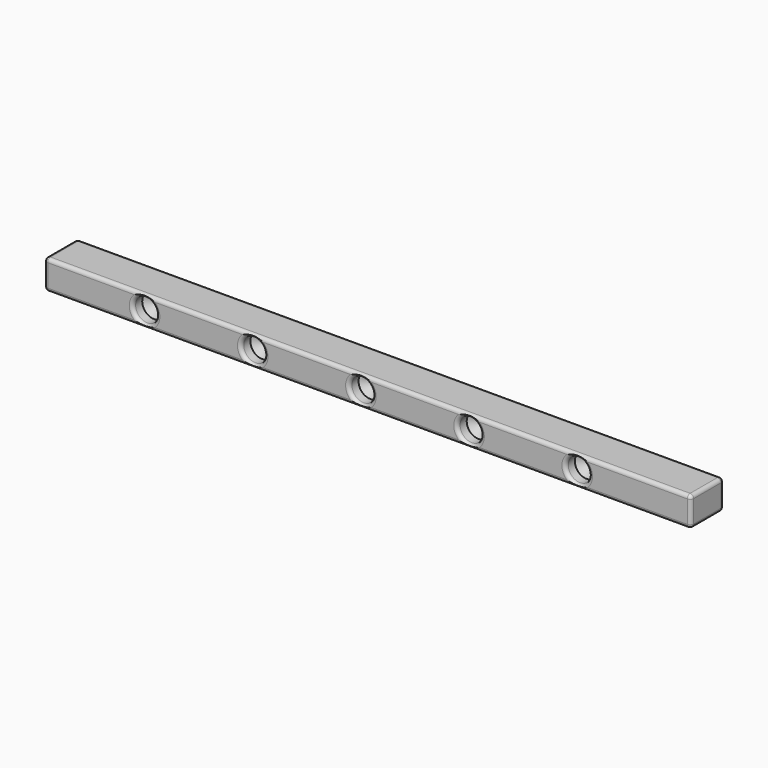
from build123d import *

# Parameters (mm, degrees)
F0_W         = 550
F0_H         = 25
F1_DEPTH     = 35
F3_D         = 20
F3_DEPTH     = 10
F3_TIP       = 6.0086061903
F4_T1_DEPTH  = 544
F4_T3_DEPTH  = 19
F4_T5_DEPTH  = 29
F4_S9_W      = 3
F4_S9_H      = 3
F4_T10_DEPTH = 3
F4_S15_W     = 3
F4_S15_H     = 3
F4_T16_DEPTH = 3
F4_S21_W     = 3
F4_S21_H     = 3
F4_T22_DEPTH = 3
F4_S27_W     = 3
F4_S27_H     = 3
F4_T28_DEPTH = 3
F4_S33_W     = 3
F4_S33_H     = 3
F4_T34_DEPTH = 3
F4_S39_W     = 3
F4_S39_H     = 3
F4_T40_DEPTH = 3
F4_S45_W     = 3
F4_S45_H     = 3
F4_T46_DEPTH = 3
F4_S51_W     = 3
F4_S51_H     = 3
F4_T52_DEPTH = 3


# Not quite as in the source:
# - a fillet or chamfer that OpenCascade refuses, or shapes differently, is made with other operations: its cross-section is extruded or revolved along the edge and cut away or added
# - a feature names something its author has since deleted; it is built from what else it names


with BuildPart() as f1:
    # F0 (on Front) → F1 (new body)
    with BuildSketch(Plane.XZ):
        with Locations((5.6565068662, -12.5)):
            Rectangle(F0_W, F0_H)
    extrude(amount=-F1_DEPTH)

    # F3
    with Locations(Plane.XZ):
        with Locations((0, -12.5), (-92, -12.5), (-184, -12.5), (92, -12.5), (184, -12.5)):
            Hole(F3_D / 2, depth=F3_DEPTH)
            with Locations((0, 0, -(F3_DEPTH + F3_TIP / 2))):  # 118° drill point
                Cone(0, F3_D / 2, F3_TIP, mode=Mode.SUBTRACT)

    # F4: fillet of radius 3 on 17 edges, made by hand

    # F4_s2 → F4_t1 (cut)
    with BuildSketch(Plane.YZ.offset(-266.3434931338)):
        with BuildLine():
            ThreePointArc((32, 0), (34.1213203436, -0.8786796564), (35, -3))
            Line((35, -3), (35, 0))
            Line((35, 0), (32, 0))
        make_face()
        with BuildLine():
            ThreePointArc((35, -22), (34.1213203436, -24.1213203436), (32, -25))
            Line((32, -25), (35, -25))
            Line((35, -25), (35, -22))
        make_face()
        with BuildLine():
            ThreePointArc((3, 0), (0.8786796564, -0.8786796564), (0, -3))
            Line((0, -3), (0, 0))
            Line((0, 0), (3, 0))
        make_face()
        with BuildLine():
            ThreePointArc((0, -22), (0.8786796564, -24.1213203436), (3, -25))
            Line((3, -25), (0, -25))
            Line((0, -25), (0, -22))
        make_face()
    extrude(amount=F4_T1_DEPTH, mode=Mode.SUBTRACT)

    # F4_s4 → F4_t3 (cut)
    with BuildSketch(Plane.XY.offset(-22)):
        with BuildLine():
            ThreePointArc((-269.3434931338, 32), (-268.4648134773, 34.1213203436), (-266.3434931338, 35))
            Line((-266.3434931338, 35), (-269.3434931338, 35))
            Line((-269.3434931338, 35), (-269.3434931338, 32))
        make_face()
        with BuildLine():
            ThreePointArc((280.6565068662, 32), (279.7778272098, 34.1213203436), (277.6565068662, 35))
            Line((277.6565068662, 35), (280.6565068662, 35))
            Line((280.6565068662, 35), (280.6565068662, 32))
        make_face()
        with BuildLine():
            ThreePointArc((280.6565068662, 3), (279.7778272098, 0.8786796564), (277.6565068662, 0))
            Line((277.6565068662, 0), (280.6565068662, 0))
            Line((280.6565068662, 0), (280.6565068662, 3))
        make_face()
        with BuildLine():
            ThreePointArc((-269.3434931338, 3), (-268.4648134773, 0.8786796564), (-266.3434931338, 0))
            Line((-266.3434931338, 0), (-269.3434931338, 0))
            Line((-269.3434931338, 0), (-269.3434931338, 3))
        make_face()
    extrude(amount=F4_T3_DEPTH, mode=Mode.SUBTRACT)

    # F4_s6 → F4_t5 (cut)
    with BuildSketch(Plane.XZ.offset(-32)):
        with BuildLine():
            ThreePointArc((280.6565068662, -22), (279.7778272098, -24.1213203436), (277.6565068662, -25))
            Line((277.6565068662, -25), (280.6565068662, -25))
            Line((280.6565068662, -25), (280.6565068662, -22))
        make_face()
        with BuildLine():
            ThreePointArc((277.6565068662, 0), (279.7778272098, -0.8786796564), (280.6565068662, -3))
            Line((280.6565068662, -3), (280.6565068662, 0))
            Line((280.6565068662, 0), (277.6565068662, 0))
        make_face()
        with BuildLine():
            ThreePointArc((-266.3434931338, 0), (-268.4648134773, -0.8786796564), (-269.3434931338, -3))
            Line((-269.3434931338, -3), (-269.3434931338, 0))
            Line((-269.3434931338, 0), (-266.3434931338, 0))
        make_face()
        with BuildLine():
            ThreePointArc((-269.3434931338, -22), (-268.4648134773, -24.1213203436), (-266.3434931338, -25))
            Line((-266.3434931338, -25), (-269.3434931338, -25))
            Line((-269.3434931338, -25), (-269.3434931338, -22))
        make_face()
    extrude(amount=F4_T5_DEPTH, mode=Mode.SUBTRACT)


with BuildPart() as f4_tool8:
    # F4_s9 → F4_t10 (new body)
    with BuildSketch(Plane.XY.offset(-3)):
        with Locations((279.1565068662, 33.5)):
            Rectangle(F4_S9_W, F4_S9_H)
    extrude(amount=F4_T10_DEPTH)

    # F4_s11 → F4_t12 (revolve, cut)
    with BuildSketch(Plane(origin=(277.6565068662, 32, -3), x_dir=(-0.7071067812, -0.7071067812, 0), z_dir=(-0.7071067812, 0.7071067812, 0))):
        with BuildLine():
            ThreePointArc((0, -3), (3, 0), (0, 3))
            Line((0, 3), (0, -3))
        make_face()
    revolve(axis=Axis((277.6565068662, 32, -3), (0, 0, 1)), mode=Mode.SUBTRACT)


with BuildPart() as f1_1:
    add(f1.part)

    # F4_t7: cut F4_tool8
    add(f4_tool8.part, mode=Mode.SUBTRACT)


with BuildPart() as f4_tool14:
    # F4_s15 → F4_t16 (new body)
    with BuildSketch(Plane.XY.offset(-3)):
        with Locations((-267.8434931338, 33.5)):
            Rectangle(F4_S15_W, F4_S15_H)
    extrude(amount=F4_T16_DEPTH)

    # F4_s17 → F4_t18 (revolve, cut)
    with BuildSketch(Plane(origin=(-266.3434931338, 32, -3), x_dir=(0.7071067812, -0.7071067812, 0), z_dir=(-0.7071067812, -0.7071067812, 0))):
        with BuildLine():
            ThreePointArc((0, -3), (3, 0), (0, 3))
            Line((0, 3), (0, -3))
        make_face()
    revolve(axis=Axis((-266.3434931338, 32, -3), (0, 0, 1)), mode=Mode.SUBTRACT)


with BuildPart() as f1_2:
    add(f1_1.part)

    # F4_t13: cut F4_tool14
    add(f4_tool14.part, mode=Mode.SUBTRACT)


with BuildPart() as f4_tool20:
    # F4_s21 → F4_t22 (new body)
    with BuildSketch(Plane.YZ.offset(-266.3434931338)):
        with Locations((33.5, -23.5)):
            Rectangle(F4_S21_W, F4_S21_H)
    extrude(amount=-F4_T22_DEPTH)

    # F4_s23 → F4_t24 (revolve, cut)
    with BuildSketch(Plane(origin=(-266.3434931338, 32, -22), x_dir=(0, -0.7071067812, 0.7071067812), z_dir=(0, -0.7071067812, -0.7071067812))):
        with BuildLine():
            ThreePointArc((0, -3), (3, 0), (0, 3))
            Line((0, 3), (0, -3))
        make_face()
    revolve(axis=Axis((-266.3434931338, 32, -22), (-1, 0, 0)), mode=Mode.SUBTRACT)


with BuildPart() as f1_3:
    add(f1_2.part)

    # F4_t19: cut F4_tool20
    add(f4_tool20.part, mode=Mode.SUBTRACT)


with BuildPart() as f4_tool26:
    # F4_s27 → F4_t28 (new body)
    with BuildSketch(Plane.YZ.offset(277.6565068662)):
        with Locations((33.5, -23.5)):
            Rectangle(F4_S27_W, F4_S27_H)
    extrude(amount=F4_T28_DEPTH)

    # F4_s29 → F4_t30 (revolve, cut)
    with BuildSketch(Plane(origin=(277.6565068662, 32, -22), x_dir=(0, -0.7071067812, 0.7071067812), z_dir=(0, 0.7071067812, 0.7071067812))):
        with BuildLine():
            ThreePointArc((0, -3), (3, 0), (0, 3))
            Line((0, 3), (0, -3))
        make_face()
    revolve(axis=Axis((277.6565068662, 32, -22), (1, 0, 0)), mode=Mode.SUBTRACT)


with BuildPart() as f1_4:
    add(f1_3.part)

    # F4_t25: cut F4_tool26
    add(f4_tool26.part, mode=Mode.SUBTRACT)


with BuildPart() as f4_tool32:
    # F4_s33 → F4_t34 (new body)
    with BuildSketch(Plane.YZ.offset(277.6565068662)):
        with Locations((1.5, -23.5)):
            Rectangle(F4_S33_W, F4_S33_H)
    extrude(amount=F4_T34_DEPTH)

    # F4_s35 → F4_t36 (revolve, cut)
    with BuildSketch(Plane(origin=(277.6565068662, 3, -22), x_dir=(0, 0.7071067812, 0.7071067812), z_dir=(0, 0.7071067812, -0.7071067812))):
        with BuildLine():
            ThreePointArc((0, -3), (3, 0), (0, 3))
            Line((0, 3), (0, -3))
        make_face()
    revolve(axis=Axis((277.6565068662, 3, -22), (1, 0, 0)), mode=Mode.SUBTRACT)


with BuildPart() as f1_5:
    add(f1_4.part)

    # F4_t31: cut F4_tool32
    add(f4_tool32.part, mode=Mode.SUBTRACT)


with BuildPart() as f4_tool38:
    # F4_s39 → F4_t40 (new body)
    with BuildSketch(Plane.XY.offset(-3)):
        with Locations((279.1565068662, 1.5)):
            Rectangle(F4_S39_W, F4_S39_H)
    extrude(amount=F4_T40_DEPTH)

    # F4_s41 → F4_t42 (revolve, cut)
    with BuildSketch(Plane(origin=(277.6565068662, 3, -3), x_dir=(-0.7071067812, 0.7071067812, 0), z_dir=(0.7071067812, 0.7071067812, 0))):
        with BuildLine():
            ThreePointArc((0, -3), (3, 0), (0, 3))
            Line((0, 3), (0, -3))
        make_face()
    revolve(axis=Axis((277.6565068662, 3, -3), (0, 0, 1)), mode=Mode.SUBTRACT)


with BuildPart() as f1_6:
    add(f1_5.part)

    # F4_t37: cut F4_tool38
    add(f4_tool38.part, mode=Mode.SUBTRACT)


with BuildPart() as f4_tool44:
    # F4_s45 → F4_t46 (new body)
    with BuildSketch(Plane.XY.offset(-3)):
        with Locations((-267.8434931338, 1.5)):
            Rectangle(F4_S45_W, F4_S45_H)
    extrude(amount=F4_T46_DEPTH)

    # F4_s47 → F4_t48 (revolve, cut)
    with BuildSketch(Plane(origin=(-266.3434931338, 3, -3), x_dir=(0.7071067812, 0.7071067812, 0), z_dir=(0.7071067812, -0.7071067812, 0))):
        with BuildLine():
            ThreePointArc((0, -3), (3, 0), (0, 3))
            Line((0, 3), (0, -3))
        make_face()
    revolve(axis=Axis((-266.3434931338, 3, -3), (0, 0, 1)), mode=Mode.SUBTRACT)


with BuildPart() as f1_7:
    add(f1_6.part)

    # F4_t43: cut F4_tool44
    add(f4_tool44.part, mode=Mode.SUBTRACT)


with BuildPart() as f4_tool50:
    # F4_s51 → F4_t52 (new body)
    with BuildSketch(Plane.YZ.offset(-266.3434931338)):
        with Locations((1.5, -23.5)):
            Rectangle(F4_S51_W, F4_S51_H)
    extrude(amount=-F4_T52_DEPTH)

    # F4_s53 → F4_t54 (revolve, cut)
    with BuildSketch(Plane(origin=(-266.3434931338, 3, -22), x_dir=(0, 0.7071067812, 0.7071067812), z_dir=(0, -0.7071067812, 0.7071067812))):
        with BuildLine():
            ThreePointArc((0, -3), (3, 0), (0, 3))
            Line((0, 3), (0, -3))
        make_face()
    revolve(axis=Axis((-266.3434931338, 3, -22), (-1, 0, 0)), mode=Mode.SUBTRACT)


with BuildPart() as f1_8:
    add(f1_7.part)

    # F4_t49: cut F4_tool50
    add(f4_tool50.part, mode=Mode.SUBTRACT)

    # F4_s55 → F4_t56 (revolve, cut)
    with BuildSketch(Plane.XY.offset(-12.5)):
        with BuildLine():
            ThreePointArc((-171, 0), (-173.1213203436, 0.8786796564), (-174, 3))
            Line((-174, 3), (-174, 0))
            Line((-174, 0), (-171, 0))
        make_face()
    revolve(axis=Axis((-184, 0, -12.5), (0, -1, 0)), mode=Mode.SUBTRACT)

    # F4_s57 → F4_t58 (revolve, cut)
    with BuildSketch(Plane.XY.offset(-12.5)):
        with BuildLine():
            ThreePointArc((-79, 0), (-81.1213203436, 0.8786796564), (-82, 3))
            Line((-82, 3), (-82, 0))
            Line((-82, 0), (-79, 0))
        make_face()
    revolve(axis=Axis((-92, 0, -12.5), (0, -1, 0)), mode=Mode.SUBTRACT)

    # F4_s59 → F4_t60 (revolve, cut)
    with BuildSketch(Plane.XY.offset(-12.5)):
        with BuildLine():
            ThreePointArc((13, 0), (10.8786796564, 0.8786796564), (10, 3))
            Line((10, 3), (10, 0))
            Line((10, 0), (13, 0))
        make_face()
    revolve(axis=Axis((0, 0, -12.5), (0, -1, 0)), mode=Mode.SUBTRACT)

    # F4_s61 → F4_t62 (revolve, cut)
    with BuildSketch(Plane.XY.offset(-12.5)):
        with BuildLine():
            ThreePointArc((105, 0), (102.8786796564, 0.8786796564), (102, 3))
            Line((102, 3), (102, 0))
            Line((102, 0), (105, 0))
        make_face()
    revolve(axis=Axis((92, 0, -12.5), (0, -1, 0)), mode=Mode.SUBTRACT)

    # F4_s63 → F4_t64 (revolve, cut)
    with BuildSketch(Plane.XY.offset(-12.5)):
        with BuildLine():
            ThreePointArc((197, 0), (194.8786796564, 0.8786796564), (194, 3))
            Line((194, 3), (194, 0))
            Line((194, 0), (197, 0))
        make_face()
    revolve(axis=Axis((184, 0, -12.5), (0, -1, 0)), mode=Mode.SUBTRACT)


solid = f1_8.part
